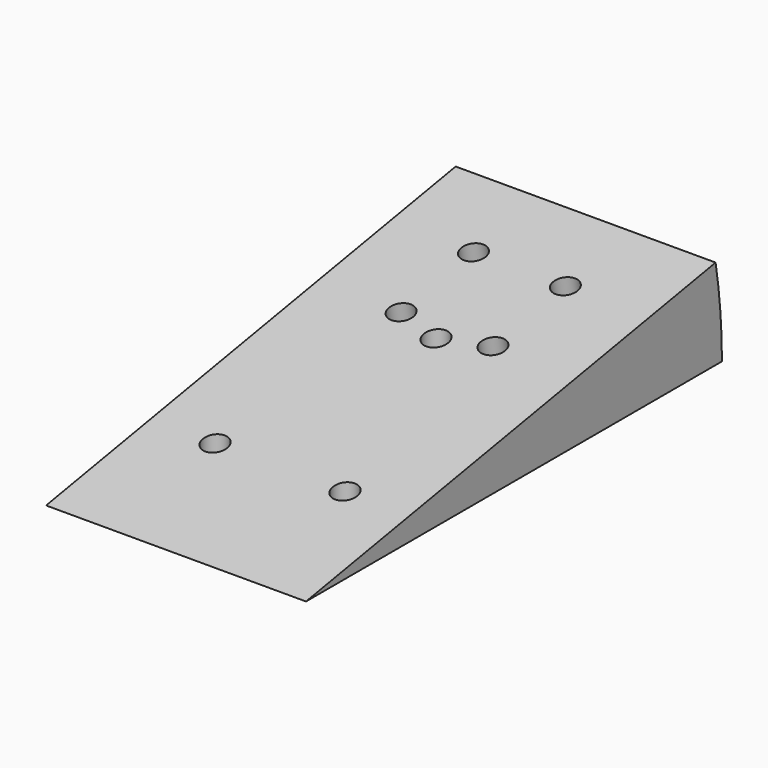
from build123d import *

# Parameters (mm, degrees)
F0_W     = 32
F0_H     = 64
F1_ANGLE = 10
F2_R     = 1.5
F3_DEPTH = 6
F4_R     = 1.5
F5_DEPTH = 8


with BuildPart() as f1:
    # F0 (on Top) → F1 (revolve)
    with BuildSketch(Plane.XY):
        Rectangle(F0_W, F0_H)
    revolve(axis=Axis((0, -32, 0), (1, 0, 0)), revolution_arc=F1_ANGLE)

    # F2 (on face) → F3 (cut)
    with BuildSketch(Plane(origin=(0, -0.9649180674, 5.4723222932), x_dir=(1, 0, 0), z_dir=(0, -0.1736481777, 0.984807753))):
        with Locations((-5.6568542495, 22.1430061531)):
            Circle(F2_R)
        with Locations((5.6568542495, 22.1430061531)):
            Circle(F2_R)
        with Locations((5.6568542495, 10.8292976541)):
            Circle(F2_R)
        with Locations((-5.6568542495, 10.8292976541)):
            Circle(F2_R)
    extrude(amount=-F3_DEPTH, mode=Mode.SUBTRACT)

    # F4 (on face) → F5 (cut)
    with BuildSketch(Plane(origin=(0, 0, 0), x_dir=(1, 0, 0), z_dir=(0, 0, -1))):
        with Locations((0, -8)):
            Circle(F4_R)
        with Locations((8, -16)):
            Circle(F4_R)
        with Locations((0, -24)):
            Circle(F4_R)
        with Locations((-8, -16)):
            Circle(F4_R)
        with Locations((-8, 16)):
            Circle(F4_R)
        with Locations((8, 16)):
            Circle(F4_R)
    extrude(amount=-F5_DEPTH, mode=Mode.SUBTRACT)


solid = f1.part
